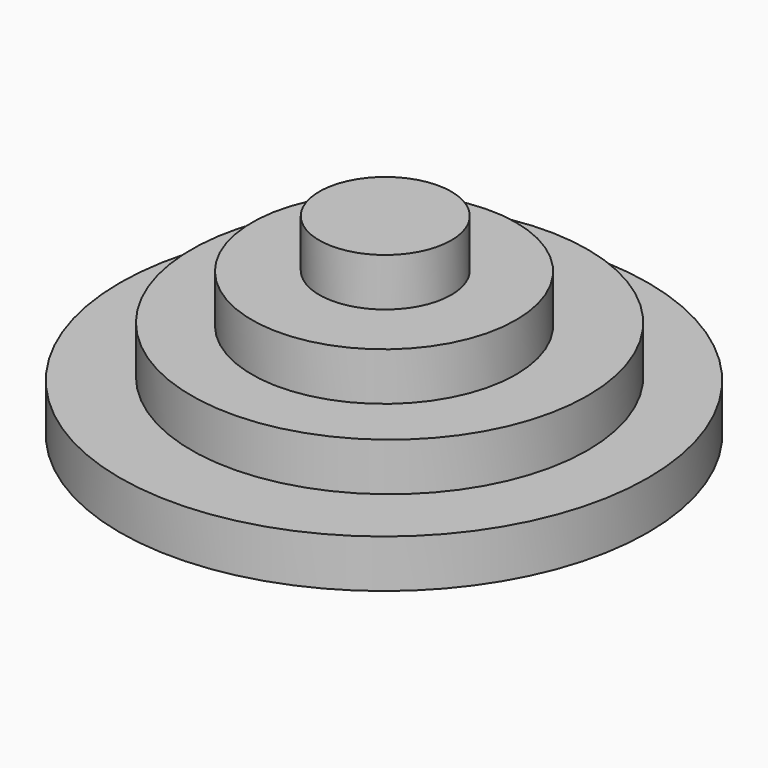
from build123d import *

# Parameters (mm, degrees)
F0_R     = 11
F1_DEPTH = 2
F2_R     = 8.25
F3_DEPTH = 2
F4_R     = 5.5
F5_DEPTH = 2
F6_R     = 2.75
F7_DEPTH = 2


# Not quite as in the source:
# - a feature names something its author has since deleted; it is built from what else it names


with BuildPart() as f1:
    # F0 (on Top) → F1 (new body)
    with BuildSketch(Plane.XY):
        Circle(F0_R)
    extrude(amount=F1_DEPTH)

    # F2 (on face) → F3 (join)
    with BuildSketch(Plane.XY.offset(2)):
        with Locations((0, 0.2906154259)):
            Circle(F2_R)
    extrude(amount=F3_DEPTH)

    # F4 (on face) → F5 (join)
    with BuildSketch(Plane.XY.offset(4)):
        Circle(F4_R)
    extrude(amount=F5_DEPTH)

    # F6 (on face) → F7 (join)
    with BuildSketch(Plane.XY.offset(6)):
        with Locations((0, 0.0671765927)):
            Circle(F6_R)
    extrude(amount=F7_DEPTH)


solid = f1.part
